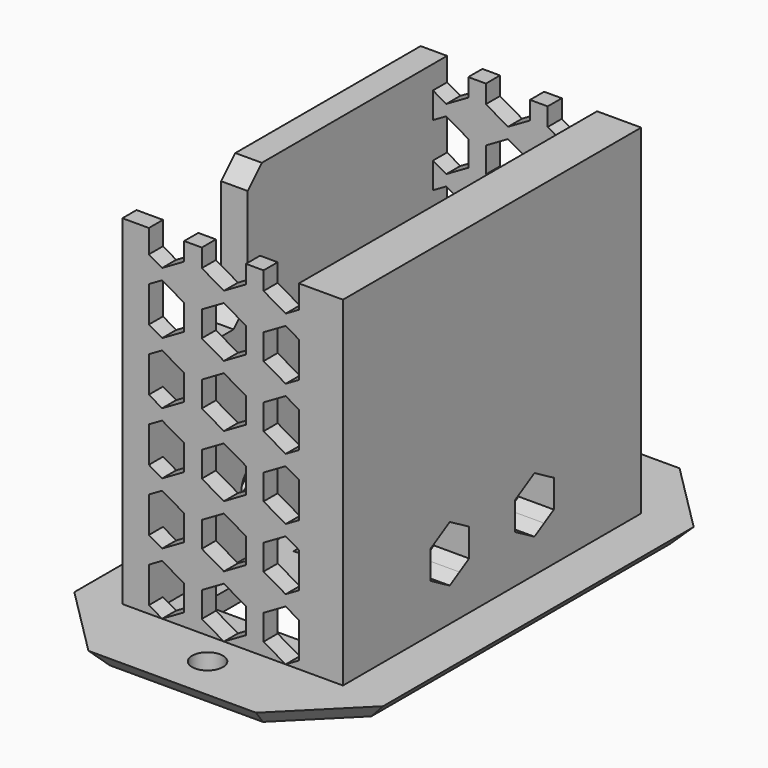
from build123d import *

# Parameters (mm, degrees)
F0_W      = 35
F0_H      = 60
F0_R      = 1.75
F0_W_2    = 14.5
F0_H_2    = 7.5
F1_DEPTH  = 2
F2_W      = 25
F2_H      = 42.25
F3_DEPTH  = 38.5
F4_R      = 2
F5_DEPTH  = 30.251
F4_W      = 12
F4_H      = 15
F6_DEPTH  = 3
F8_DEPTH  = 42.25
F9_SIZE   = 8
F10_SIZE  = 1.99999
F11_SIZE  = 2
F12_DEPTH = 1
F13_START = -21
F13_DEPTH = 4


# Not quite as in the source:
# - a fillet or chamfer is up to 0.001 mm smaller than in the source, because OpenCascade refuses the exact size


with BuildPart() as f1:
    # F0 (on Top) → F1 (new body)
    with BuildSketch(Plane.XY):
        Rectangle(F0_W, F0_H)
        with Locations((0, -25)):
            Circle(F0_R, mode=Mode.SUBTRACT)
        with Locations((0, -13)):
            Rectangle(F0_W_2, F0_H_2, mode=Mode.SUBTRACT)
        Rectangle(F0_W_2, F0_H_2, mode=Mode.SUBTRACT)
        with Locations((0, 13)):
            Rectangle(F0_W_2, F0_H_2, mode=Mode.SUBTRACT)
        with Locations((0, 25)):
            Circle(F0_R, mode=Mode.SUBTRACT)
    extrude(amount=F1_DEPTH)

    # F2 (on face) → F3 (join)
    with BuildSketch(Plane.XY.offset(2)):
        with Locations((-0.25, 0)):
            Rectangle(F2_W, F2_H)
        Polygon((-9.75, 19.125), (7.25, 19.125), (7.25, 16.75), (7.25, 9.25), (7.25, 3.75), (7.25, -3.75), (7.25, -9.25), (7.25, -16.75), (7.25, -19.125), (-9.75, -19.125), align=None, mode=Mode.SUBTRACT)
    extrude(amount=F3_DEPTH)

    # F4 (on face) → F5 (cut, through all)
    with BuildSketch(Plane(origin=(-12.75, 0, 0), x_dir=(0, -1, 0), z_dir=(-1, 0, 0))):
        with Locations((-6, 9)):
            Circle(F4_R)
        with Locations((6, 9)):
            Circle(F4_R)
    extrude(amount=-F5_DEPTH, mode=Mode.SUBTRACT)

    # F4 (on face) → F6 (cut, through all)
    with BuildSketch(Plane(origin=(-12.75, 0, 0), x_dir=(0, -1, 0), z_dir=(-1, 0, 0))):
        with Locations((13.125, 33)):
            Rectangle(F4_W, F4_H)
    extrude(amount=-F6_DEPTH, mode=Mode.SUBTRACT)

    # F7 (on face) → F8 (cut, through all)
    with BuildSketch(Plane.XZ.offset(21.125)):
        Polygon((-5.75, 40.5), (-9.75, 40.5), (-9.75, 37.8660254038), (-8.25, 37), (-5.75, 38.443375673), align=None)
        Polygon((1.25, 40.5), (-3.75, 40.5), (-3.75, 38.443375673), (-1.25, 37), (1.25, 38.443375673), align=None)
        Polygon((7.25, 37.8660254038), (7.25, 40.5), (3.25, 40.5), (3.25, 38.443375673), (5.75, 37), align=None)
        Polygon((7.25, 30.8660254038), (7.25, 34.9074772881), (5.75, 35.7735026919), (3.25, 34.3301270189), (3.25, 31.443375673), (5.75, 30), align=None)
        Polygon((1.25, 34.3301270189), (-1.25, 35.7735026919), (-3.75, 34.3301270189), (-3.75, 31.443375673), (-1.25, 30), (1.25, 31.443375673), align=None)
        Polygon((-9.75, 34.9074772881), (-9.75, 30.8660254038), (-8.25, 30), (-5.75, 31.443375673), (-5.75, 34.3301270189), (-8.25, 35.7735026919), align=None)
        Polygon((-9.75, 27.9074772881), (-9.75, 23.8660254038), (-8.25, 23), (-5.75, 24.443375673), (-5.75, 27.3301270189), (-8.25, 28.7735026919), align=None)
        Polygon((1.25, 27.3301270189), (-1.25, 28.7735026919), (-3.75, 27.3301270189), (-3.75, 24.443375673), (-1.25, 23), (1.25, 24.443375673), align=None)
        Polygon((5.75, 23), (7.25, 23.8660254038), (7.25, 27.9074772881), (5.75, 28.7735026919), (3.25, 27.3301270189), (3.25, 24.443375673), align=None)
        Polygon((5.75, 16), (7.25, 16.8660254038), (7.25, 20.9074772881), (5.75, 21.7735026919), (3.25, 20.3301270189), (3.25, 17.443375673), align=None)
        Polygon((1.25, 20.3301270189), (-1.25, 21.7735026919), (-3.75, 20.3301270189), (-3.75, 17.443375673), (-1.25, 16), (1.25, 17.443375673), align=None)
        Polygon((-9.75, 20.9074772881), (-9.75, 16.8660254038), (-8.25, 16), (-5.75, 17.443375673), (-5.75, 20.3301270189), (-8.25, 21.7735026919), align=None)
        Polygon((-9.75, 13.9074772881), (-9.75, 9.8660254038), (-8.25, 9), (-5.75, 10.443375673), (-5.75, 13.3301270189), (-8.25, 14.7735026919), align=None)
        Polygon((1.25, 13.3301270189), (-1.25, 14.7735026919), (-3.75, 13.3301270189), (-3.75, 10.443375673), (-1.25, 9), (1.25, 10.443375673), align=None)
        Polygon((5.75, 9), (7.25, 9.8660254038), (7.25, 13.9074772881), (5.75, 14.7735026919), (3.25, 13.3301270189), (3.25, 10.443375673), align=None)
        Polygon((3.25, 3.443375673), (5.75, 2), (7.25, 2.8660254038), (7.25, 6.9074772881), (5.75, 7.7735026919), (3.25, 6.3301270189), align=None)
        Polygon((-3.75, 3.443375673), (-1.25, 2), (1.25, 3.443375673), (1.25, 6.3301270189), (-1.25, 7.7735026919), (-3.75, 6.3301270189), align=None)
        Polygon((-5.75, 6.3301270189), (-8.25, 7.7735026919), (-9.75, 6.9074772881), (-9.75, 2.8660254038), (-8.25, 2), (-5.75, 3.443375673), align=None)
    extrude(amount=-F8_DEPTH, mode=Mode.SUBTRACT)

    # F9
    f9_edges = [f1.edges().sort_by_distance(p)[0] for p in [
        (-17.5, -30, 1),
        (17.5, -30, 1),
        (17.5, 30, 1),
        (-17.5, 30, 1),
    ]]
    chamfer(f9_edges, length=F9_SIZE)

    # F10 (size 2 in the source; OpenCascade refuses exactly that, so slightly less here)
    f10_edges = [f1.edges().sort_by_distance(p)[0] for p in [
        (-13.5, 26, 0),
        (0, 30, 0),
        (13.5, 26, 0),
        (17.5, 0, 0),
        (13.5, -26, 0),
        (0, -30, 0),
        (-13.5, -26, 0),
        (-17.5, 0, 0),
    ]]
    chamfer(f10_edges, length=F10_SIZE)

    # F11
    f11_edges = [f1.edges().sort_by_distance(p)[0] for p in [
        (7.25, 6.5, 2),
        (7.25, -6.5, 2),
        (-11.25, -7.125, 25.5),
        (-11.25, -19.125, 25.5),
        (-11.25, -7.125, 40.5),
    ]]
    chamfer(f11_edges, length=F11_SIZE)

    # F4 (on face) → F12 (cut)
    with BuildSketch(Plane(origin=(-12.75, 0, 0), x_dir=(0, -1, 0), z_dir=(-1, 0, 0))):
        with BuildLine():
            ThreePointArc((-4.6250000224, 6.6184301267), (-3.6184301461, 7.6249999888), (-3.25, 9))
            ThreePointArc((-3.25, 9), (-3.6184301267, 10.3749999777), (-4.6249999554, 11.3815698346))
            ThreePointArc((-4.6249999554, 11.3815698346), (-5.9999999613, 11.75), (-7.3749999776, 11.3815698733))
            ThreePointArc((-7.3749999776, 11.3815698733), (-8.3815698539, 10.3750000112), (-8.75, 9))
            ThreePointArc((-8.75, 9), (-8.3815698836, 7.6250000402), (-7.3750000803, 6.618430186))
            ThreePointArc((-7.3750000803, 6.618430186), (-6.0000000593, 6.25), (-4.6250000224, 6.6184301267))
        make_face()
        with Locations((-6, 9)):
            Circle(F4_R, mode=Mode.SUBTRACT)
        with BuildLine():
            ThreePointArc((7.3750000653, 6.6184301773), (8.3815698793, 7.6250000327), (8.75, 9))
            ThreePointArc((8.75, 9), (8.3815698836, 10.3749999598), (7.3750000803, 11.381569814))
            ThreePointArc((7.3750000803, 11.381569814), (6.0000000733, 11.75), (4.6250000466, 11.3815698873))
            ThreePointArc((4.6250000466, 11.3815698873), (3.6184301531, 10.3750000233), (3.25, 9))
            ThreePointArc((3.25, 9), (3.6184301461, 7.6249999888), (4.6250000224, 6.6184301267))
            ThreePointArc((4.6250000224, 6.6184301267), (6.0000000507, 6.25), (7.3750000653, 6.6184301773))
        make_face()
        with Locations((6, 9)):
            Circle(F4_R, mode=Mode.SUBTRACT)
    extrude(amount=-F12_DEPTH, mode=Mode.SUBTRACT)

    # F4 (on face) → F13 (cut)
    with BuildSketch(Plane(origin=(-12.75, 0, 0), x_dir=(0, -1, 0), z_dir=(-1, 0, 0)).offset(F13_START)):
        with BuildLine():
            ThreePointArc((7.3750000653, 6.6184301773), (8.3815698793, 7.6250000327), (8.75, 9))
            ThreePointArc((8.75, 9), (8.3815698836, 10.3749999598), (7.3750000803, 11.381569814))
            ThreePointArc((7.3750000803, 11.381569814), (6.0000000733, 11.75), (4.6250000466, 11.3815698873))
            ThreePointArc((4.6250000466, 11.3815698873), (3.6184301531, 10.3750000233), (3.25, 9))
            ThreePointArc((3.25, 9), (3.6184301461, 7.6249999888), (4.6250000224, 6.6184301267))
            ThreePointArc((4.6250000224, 6.6184301267), (6.0000000507, 6.25), (7.3750000653, 6.6184301773))
        make_face()
        with Locations((6, 9)):
            Circle(F4_R, mode=Mode.SUBTRACT)
        with BuildLine():
            ThreePointArc((-4.6250000224, 6.6184301267), (-3.6184301461, 7.6249999888), (-3.25, 9))
            ThreePointArc((-3.25, 9), (-3.6184301267, 10.3749999777), (-4.6249999554, 11.3815698346))
            ThreePointArc((-4.6249999554, 11.3815698346), (-5.9999999613, 11.75), (-7.3749999776, 11.3815698733))
            ThreePointArc((-7.3749999776, 11.3815698733), (-8.3815698539, 10.3750000112), (-8.75, 9))
            ThreePointArc((-8.75, 9), (-8.3815698836, 7.6250000402), (-7.3750000803, 6.618430186))
            ThreePointArc((-7.3750000803, 6.618430186), (-6.0000000593, 6.25), (-4.6250000224, 6.6184301267))
        make_face()
        with Locations((-6, 9)):
            Circle(F4_R, mode=Mode.SUBTRACT)
        with Locations((-6, 9)):
            Circle(F4_R)
        with Locations((6, 9)):
            Circle(F4_R)
        with BuildLine():
            ThreePointArc((-4.6249999554, 11.3815698346), (-3.6184301267, 10.3749999777), (-3.25, 9))
            Line((-3.25, 9), (-3.25, 10.5877132403))
            Line((-3.25, 10.5877132403), (-4.6249999554, 11.3815698346))
        make_face()
        with BuildLine():
            Line((6, 5.8245735195), (7.3750000653, 6.6184301773))
            ThreePointArc((7.3750000653, 6.6184301773), (6.0000000507, 6.25), (4.6250000224, 6.6184301267))
            Line((4.6250000224, 6.6184301267), (6, 5.8245735195))
        make_face()
        with BuildLine():
            Line((8.75, 7.4122867597), (8.75, 9))
            ThreePointArc((8.75, 9), (8.3815698793, 7.6250000327), (7.3750000653, 6.6184301773))
            Line((7.3750000653, 6.6184301773), (8.75, 7.4122867597))
        make_face()
        with BuildLine():
            Line((-3.25, 7.4122867597), (-3.25, 9))
            ThreePointArc((-3.25, 9), (-3.6184301461, 7.6249999888), (-4.6250000224, 6.6184301267))
            Line((-4.6250000224, 6.6184301267), (-3.25, 7.4122867597))
        make_face()
        with BuildLine():
            ThreePointArc((7.3750000803, 11.381569814), (8.3815698836, 10.3749999598), (8.75, 9))
            Line((8.75, 9), (8.75, 10.5877132403))
            Line((8.75, 10.5877132403), (7.3750000803, 11.381569814))
        make_face()
        with BuildLine():
            Line((3.25, 7.4122867597), (4.6250000224, 6.6184301267))
            ThreePointArc((4.6250000224, 6.6184301267), (3.6184301461, 7.6249999888), (3.25, 9))
            Line((3.25, 9), (3.25, 7.4122867597))
        make_face()
        with BuildLine():
            ThreePointArc((-7.3749999776, 11.3815698733), (-5.9999999613, 11.75), (-4.6249999554, 11.3815698346))
            Line((-4.6249999554, 11.3815698346), (-6, 12.1754264805))
            Line((-6, 12.1754264805), (-7.3749999776, 11.3815698733))
        make_face()
        with BuildLine():
            Line((-6, 5.8245735195), (-4.6250000224, 6.6184301267))
            ThreePointArc((-4.6250000224, 6.6184301267), (-6.0000000593, 6.25), (-7.3750000803, 6.618430186))
            Line((-7.3750000803, 6.618430186), (-6, 5.8245735195))
        make_face()
        with BuildLine():
            ThreePointArc((-8.75, 9), (-8.3815698539, 10.3750000112), (-7.3749999776, 11.3815698733))
            Line((-7.3749999776, 11.3815698733), (-8.75, 10.5877132403))
            Line((-8.75, 10.5877132403), (-8.75, 9))
        make_face()
        with BuildLine():
            ThreePointArc((4.6250000466, 11.3815698873), (6.0000000733, 11.75), (7.3750000803, 11.381569814))
            Line((7.3750000803, 11.381569814), (6, 12.1754264805))
            Line((6, 12.1754264805), (4.6250000466, 11.3815698873))
        make_face()
        with BuildLine():
            ThreePointArc((3.25, 9), (3.6184301531, 10.3750000233), (4.6250000466, 11.3815698873))
            Line((4.6250000466, 11.3815698873), (3.25, 10.5877132403))
            Line((3.25, 10.5877132403), (3.25, 9))
        make_face()
        with BuildLine():
            Line((-8.75, 7.4122867597), (-7.3750000803, 6.618430186))
            ThreePointArc((-7.3750000803, 6.618430186), (-8.3815698836, 7.6250000402), (-8.75, 9))
            Line((-8.75, 9), (-8.75, 7.4122867597))
        make_face()
    extrude(amount=-F13_DEPTH, mode=Mode.SUBTRACT)


solid = f1.part
